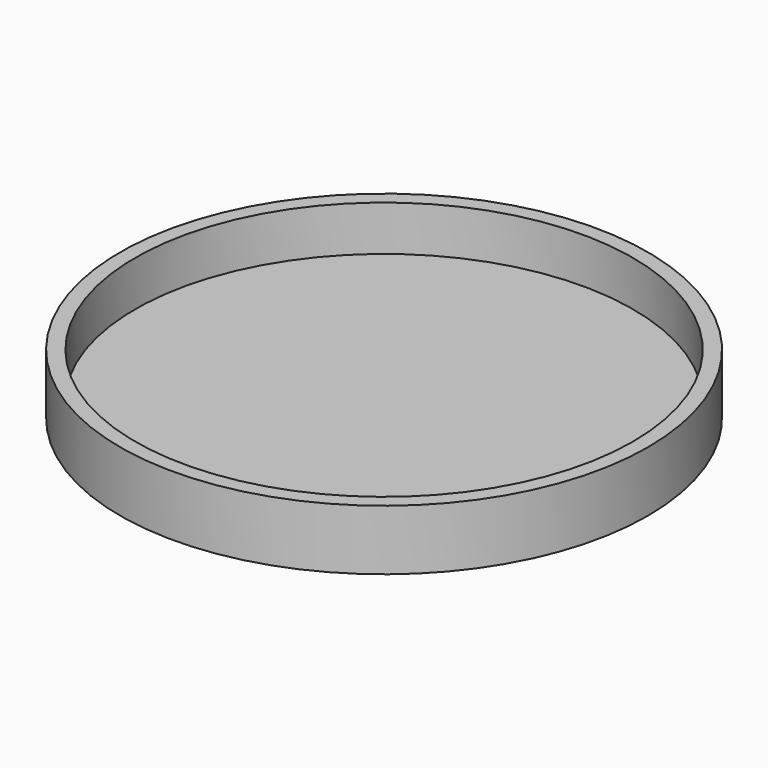
from build123d import *

# Parameters (mm, degrees)
F0_R     = 17.5
F1_DEPTH = 4
F2_R     = 16.5
F3_DEPTH = 3


# Not quite as in the source:
# - the program builds the solid bodies; features that only make, move or delete a surface that nothing else refers to are left out


with BuildPart() as f1:
    # F0 (on Top) → F1 (new body)
    with BuildSketch(Plane.XY):
        Circle(F0_R)
    extrude(amount=F1_DEPTH)

    # F2 (on face) → F3 (cut)
    with BuildSketch(Plane.XY.offset(4)):
        Circle(F2_R)
    extrude(amount=-F3_DEPTH, mode=Mode.SUBTRACT)


solid = f1.part
